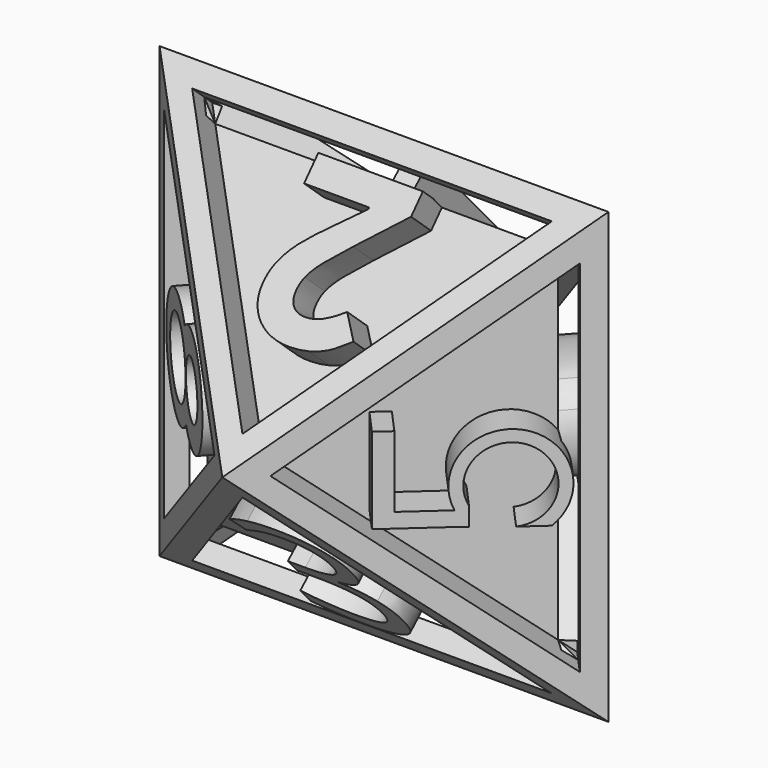
from build123d import *

# Parameters (mm, degrees)
F0_W      = 20
F0_H      = 20
F1_FACE_W = 20
F1_FACE_H = 20
F11_DEPTH = 1.5
F12_DEPTH = 1.5
F13_DEPTH = 1.5
F14_DEPTH = 1.5
F7_R      = 1.2292733426
F15_DEPTH = 1.5
F16_DEPTH = 1.5
F17_DEPTH = 1.5
F18_DEPTH = 1
F19_DEPTH = 1


# Not quite as in the source:
# - an extrude whose draft closes it to a point is written as a loft to that point
# - a feature names something its author has since deleted; it is built from what else it names


with BuildPart() as f1:
    # F0 (on Front) → F1 section 0
    with BuildSketch(Plane.XZ, mode=Mode.PRIVATE) as f1_s0:
        with Locations((-8.0479989899, 1.5718473494)):
            Rectangle(F0_W, F0_H)
    loft([f1_s0.sketch, Vertex(-8.0479989899, -9.004040443, 1.5718473494)], ruled=True)

    # F1_face (on face) → F2 section 0
    with BuildSketch(Plane(origin=(-8.0479989899, 0, 1.5718473494), x_dir=(1, 0, 0), z_dir=(0, 1, 0)), mode=Mode.PRIVATE) as f2_s0:
        Rectangle(F1_FACE_W, F1_FACE_H)
    loft([f2_s0.sketch, Vertex(-8.0479989899, 9.004040443, 1.5718473494)], ruled=True)

    # F8 (on face) → F11 (cut)
    with BuildSketch(Plane(origin=(0, -5.7542277794, 5.1811299644), x_dir=(1, 0, 0), z_dir=(0, -0.7431448255, 0.6691306064))):
        Polygon((-16.0589551992, 7.5995584789), (-8.0479989899, -3.1802463917), (-0.0370427807, 7.5995584789), align=None)
        with BuildLine():
            Line((-10.1255093079, 5.8311121626), (-10.1255093079, 7.0160687901))
            Line((-10.1255093079, 7.0160687901), (-5.470218449, 7.0160687901))
            Line((-5.470218449, 7.0160687901), (-5.470218449, 6.0366212456))
            Line((-5.470218449, 6.0366212456), (-7.1419838263, 4.3473657335))
            add(Edge.make_bspline(
                [(-7.1419838263, 4.3473657335), (-7.8853145521, 3.586544873), (-8.1126863035, 3.2928563608)],
                knots=[0, 0, 0, 1, 1, 1], degree=2))
            add(Edge.make_bspline(
                [(-8.1126863035, 3.2928563608), (-8.3400580549, 2.9991678486), (-8.4406263295, 2.7484759175)],
                knots=[0, 0, 0, 1, 1, 1], degree=2))
            add(Edge.make_bspline(
                [(-8.4406263295, 2.7484759175), (-8.5411946042, 2.4977839865), (-8.5411946042, 2.2296019207)],
                knots=[0, 0, 0, 1, 1, 1], degree=2))
            add(Edge.make_bspline(
                [(-8.5411946042, 2.2296019207), (-8.5411946042, 1.8287863333), (-8.3196528977, 1.6327510733)],
                knots=[0, 0, 0, 1, 1, 1], degree=2))
            add(Edge.make_bspline(
                [(-8.3196528977, 1.6327510733), (-8.0981111912, 1.4367158133), (-7.7293608508, 1.4367158133)],
                knots=[0, 0, 0, 1, 1, 1], degree=2))
            add(Edge.make_bspline(
                [(-7.7293608508, 1.4367158133), (-7.3431203756, 1.4367158133), (-6.9787425689, 1.614532183)],
                knots=[0, 0, 0, 1, 1, 1], degree=2))
            add(Edge.make_bspline(
                [(-6.9787425689, 1.614532183), (-6.6143647621, 1.7923485527), (-6.2179217084, 2.1202885787)],
                knots=[0, 0, 0, 1, 1, 1], degree=2))
            Line((-6.2179217084, 2.1202885787), (-5.4527283143, 1.2137165955))
            add(Edge.make_bspline(
                [(-5.4527283143, 1.2137165955), (-5.9439095977, 0.7939533622), (-6.2674770901, 0.6212382818)],
                knots=[0, 0, 0, 1, 1, 1], degree=2))
            add(Edge.make_bspline(
                [(-6.2674770901, 0.6212382818), (-6.5910445825, 0.4485232014), (-6.9736412796, 0.3552424829)],
                knots=[0, 0, 0, 1, 1, 1], degree=2))
            add(Edge.make_bspline(
                [(-6.9736412796, 0.3552424829), (-7.3562379767, 0.2619617643), (-7.8299291254, 0.2619617643)],
                knots=[0, 0, 0, 1, 1, 1], degree=2))
            add(Edge.make_bspline(
                [(-7.8299291254, 0.2619617643), (-8.4537439306, 0.2619617643), (-8.931807613, 0.4893335157)],
                knots=[0, 0, 0, 1, 1, 1], degree=2))
            add(Edge.make_bspline(
                [(-8.931807613, 0.4893335157), (-9.4098712955, 0.7167052671), (-9.6744095832, 1.1269946775)],
                knots=[0, 0, 0, 1, 1, 1], degree=2))
            add(Edge.make_bspline(
                [(-9.6744095832, 1.1269946775), (-9.9389478709, 1.5372840879), (-9.9389478709, 2.0649031521)],
                knots=[0, 0, 0, 1, 1, 1], degree=2))
            add(Edge.make_bspline(
                [(-9.9389478709, 2.0649031521), (-9.9389478709, 2.5254766998), (-9.7771641247, 2.9284785541)],
                knots=[0, 0, 0, 1, 1, 1], degree=2))
            add(Edge.make_bspline(
                [(-9.7771641247, 2.9284785541), (-9.6153803785, 3.3314804083), (-9.2757802626, 3.7548874198)],
                knots=[0, 0, 0, 1, 1, 1], degree=2))
            add(Edge.make_bspline(
                [(-9.2757802626, 3.7548874198), (-8.9361801467, 4.1782944312), (-8.0806210565, 4.9624354713)],
                knots=[0, 0, 0, 1, 1, 1], degree=2))
            Line((-8.0806210565, 4.9624354713), (-7.223604455, 5.7684391798))
            Line((-7.223604455, 5.7684391798), (-7.223604455, 5.8311121626))
            Line((-7.223604455, 5.8311121626), (-10.1255093079, 5.8311121626))
        make_face(mode=Mode.SUBTRACT)
    extrude(amount=-F11_DEPTH, mode=Mode.SUBTRACT)

    # F9 (on face) → F12 (cut)
    with BuildSketch(Plane(origin=(0.8739806721, -0.9706538721, 0), x_dir=(0.7431448255, 0.6691306064, 0), z_dir=(0.6691306064, -0.7431448255, 0))):
        Polygon((0.45061945, 9.5828035587), (-10.3291854207, 1.5718473494), (0.45061945, -6.4391088599), align=None)
        with BuildLine():
            Line((-6.7914770916, -0.6216760376), (-6.7914770916, 3.1999400918))
            Line((-6.7914770916, 3.1999400918), (-6.0100099072, 3.1999400918))
            Line((-6.0100099072, 3.1999400918), (-6.0100099072, 0.0335111318))
            Line((-6.0100099072, 0.0335111318), (-3.9149023546, 0.0335111318))
            ThreePointArc((-3.9149023546, 0.0335111318), (-1.5046868703, 3.1151424708), (-0.5219964927, -0.6716648932))
            Line((-0.5219964927, -0.6716648932), (-1.7677578144, -0.6716648932))
            ThreePointArc((-1.7677578144, -0.6716648932), (-1.1781497358, 2.4500116664), (-3.408615146, 0.1878166521))
            Line((-3.408615146, 0.1878166521), (-3.408615146, -0.6312971566))
            Line((-3.408615146, -0.6312971566), (-3.682563547, -0.6216760376))
            Line((-3.682563547, -0.6216760376), (-6.7914770916, -0.6216760376))
        make_face(mode=Mode.SUBTRACT)
    extrude(amount=-F12_DEPTH, mode=Mode.SUBTRACT)

    # F10 (on face) → F13 (cut)
    with BuildSketch(Plane(origin=(0, -4.1909911743, -3.7735854029), x_dir=(1, 0, 0), z_dir=(0, -0.7431448255, -0.6691306064))):
        Polygon((-0.0370427807, -5.2633380306), (-8.0479989899, 5.51646684), (-16.0589551992, -5.2633380306), align=None)
        with BuildLine():
            add(Edge.make_bspline(
                [(-6.2778853712, 2.3209247428), (-5.6446293929, 1.7983598502), (-5.6446293929, 0.8870890521)],
                knots=[0, 0, 0, 1, 1, 1], degree=2))
            add(Edge.make_bspline(
                [(-5.6446293929, 0.8870890521), (-5.6446293929, 0.1354193543), (-6.0659419747, -0.3416678055)],
                knots=[0, 0, 0, 1, 1, 1], degree=2))
            add(Edge.make_bspline(
                [(-6.0659419747, -0.3416678055), (-6.4872545565, -0.8187549653), (-7.2595179446, -0.9800722064)],
                knots=[0, 0, 0, 1, 1, 1], degree=2))
            Line((-7.2595179446, -0.9800722064), (-7.2595179446, -1.022975728))
            add(Edge.make_bspline(
                [(-7.2595179446, -1.022975728), (-6.3156404702, -1.1396733066), (-5.8600050712, -1.6227669594)],
                knots=[0, 0, 0, 1, 1, 1], degree=2))
            add(Edge.make_bspline(
                [(-5.8600050712, -1.6227669594), (-5.4043696722, -2.1058606123), (-5.4043696722, -2.8884208456)],
                knots=[0, 0, 0, 1, 1, 1], degree=2))
            add(Edge.make_bspline(
                [(-5.4043696722, -2.8884208456), (-5.4043696722, -4.0090608289), (-6.1817814829, -4.6131424125)],
                knots=[0, 0, 0, 1, 1, 1], degree=2))
            add(Edge.make_bspline(
                [(-6.1817814829, -4.6131424125), (-6.9591932937, -5.2172239962), (-8.3904547731, -5.2172239962)],
                knots=[0, 0, 0, 1, 1, 1], degree=2))
            add(Edge.make_bspline(
                [(-8.3904547731, -5.2172239962), (-9.0134139062, -5.2172239962), (-9.5308303763, -5.1228362487)],
                knots=[0, 0, 0, 1, 1, 1], degree=2))
            add(Edge.make_bspline(
                [(-9.5308303763, -5.1228362487), (-10.0482468464, -5.0284485013), (-10.5356308513, -4.7933372031)],
                knots=[0, 0, 0, 1, 1, 1], degree=2))
            Line((-10.5356308513, -4.7933372031), (-10.5356308513, -3.945563617))
            add(Edge.make_bspline(
                [(-10.5356308513, -3.945563617), (-10.0259370151, -4.1978363238), (-9.4493136853, -4.3291210998)],
                knots=[0, 0, 0, 1, 1, 1], degree=2))
            add(Edge.make_bspline(
                [(-9.4493136853, -4.3291210998), (-8.8726903555, -4.4604058758), (-8.3578480967, -4.4604058758)],
                knots=[0, 0, 0, 1, 1, 1], degree=2))
            add(Edge.make_bspline(
                [(-8.3578480967, -4.4604058758), (-6.3259373154, -4.4604058758), (-6.3259373154, -2.8678271553)],
                knots=[0, 0, 0, 1, 1, 1], degree=2))
            add(Edge.make_bspline(
                [(-6.3259373154, -2.8678271553), (-6.3259373154, -1.4399979576), (-8.5672172819, -1.4399979576)],
                knots=[0, 0, 0, 1, 1, 1], degree=2))
            Line((-8.5672172819, -1.4399979576), (-9.3394806701, -1.4399979576))
            Line((-9.3394806701, -1.4399979576), (-9.3394806701, -0.6745991329))
            Line((-9.3394806701, -0.6745991329), (-8.5569204368, -0.6745991329))
            add(Edge.make_bspline(
                [(-8.5569204368, -0.6745991329), (-7.6405012161, -0.6745991329), (-7.1042071966, -0.2695898893)],
                knots=[0, 0, 0, 1, 1, 1], degree=2))
            add(Edge.make_bspline(
                [(-7.1042071966, -0.2695898893), (-6.567913177, 0.1354193543), (-6.567913177, 0.8544823757)],
                knots=[0, 0, 0, 1, 1, 1], degree=2))
            add(Edge.make_bspline(
                [(-6.567913177, 0.8544823757), (-6.567913177, 1.4276734238), (-6.961767505, 1.7554563286)],
                knots=[0, 0, 0, 1, 1, 1], degree=2))
            add(Edge.make_bspline(
                [(-6.961767505, 1.7554563286), (-7.3556218329, 2.0832392333), (-8.0317813328, 2.0832392333)],
                knots=[0, 0, 0, 1, 1, 1], degree=2))
            add(Edge.make_bspline(
                [(-8.0317813328, 2.0832392333), (-8.5466235916, 2.0832392333), (-9.0022589906, 1.943373753)],
                knots=[0, 0, 0, 1, 1, 1], degree=2))
            add(Edge.make_bspline(
                [(-9.0022589906, 1.943373753), (-9.4578943896, 1.8035082727), (-10.0430984238, 1.4276734238)],
                knots=[0, 0, 0, 1, 1, 1], degree=2))
            Line((-10.0430984238, 1.4276734238), (-10.4927273298, 2.0283227257))
            add(Edge.make_bspline(
                [(-10.4927273298, 2.0283227257), (-10.0104917474, 2.4093059972), (-9.3806680508, 2.6263978164)],
                knots=[0, 0, 0, 1, 1, 1], degree=2))
            add(Edge.make_bspline(
                [(-9.3806680508, 2.6263978164), (-8.7508443542, 2.8434896355), (-8.0523750232, 2.8434896355)],
                knots=[0, 0, 0, 1, 1, 1], degree=2))
            add(Edge.make_bspline(
                [(-8.0523750232, 2.8434896355), (-6.9111413495, 2.8434896355), (-6.2778853712, 2.3209247428)],
                knots=[0, 0, 0, 1, 1, 1], degree=2))
        make_face(mode=Mode.SUBTRACT)
    extrude(amount=-F13_DEPTH, mode=Mode.SUBTRACT)

    # F7 (on face) → F14 (cut)
    with BuildSketch(Plane(origin=(-8.0807346952, -8.9745650815, 0), x_dir=(0.7431448255, -0.6691306064, 0), z_dir=(-0.6691306064, -0.7431448255, 0))):
        Polygon((-12.4122770596, -6.4391088599), (-1.632472189, 1.5718473494), (-12.4122770596, 9.5828035587), align=None)
        with BuildLine():
            ThreePointArc((-8.0010479185, 3.3852743433), (-4.2277937132, 1.7916034584), (-7.7158939093, -0.3555786971))
            ThreePointArc((-7.7158939093, -0.3555786971), (-11.95616225, 1.2024931008), (-8.0010479185, 3.3852743433))
        make_face(mode=Mode.SUBTRACT)
        with BuildLine():
            ThreePointArc((-7.835039689, 1.3912107131), (-7.8362300165, 1.4537861947), (-7.8397992768, 1.516271138))
            ThreePointArc((-7.8397992768, 1.516271138), (-11.1246308448, 1.3286352316), (-7.835039689, 1.3912107131))
        make_face()
    extrude(amount=-F14_DEPTH, mode=Mode.SUBTRACT)

    # F7 (on face) → F15 (cut)
    with BuildSketch(Plane(origin=(-8.0807346952, -8.9745650815, 0), x_dir=(0.7431448255, -0.6691306064, 0), z_dir=(-0.6691306064, -0.7431448255, 0))):
        with Locations((-6.5249288455, 1.616499736)):
            Circle(F7_R)
    extrude(amount=-F15_DEPTH, mode=Mode.SUBTRACT)

    # F4 (on face) → F16 (cut)
    with BuildSketch(Plane(origin=(0.8739806721, 0.9706538721, 0), x_dir=(-0.7431448255, 0.6691306064, 0), z_dir=(0.6691306064, 0.7431448255, 0))):
        Polygon((-0.45061945, -6.4391088599), (10.3291854207, 1.5718473494), (-0.45061945, 9.5828035587), align=None)
        with BuildLine():
            add(Edge.make_bspline(
                [(1.6306424047, 3.545827145), (2.2208165521, 3.8140285075), (3.053617849, 3.8140285075)],
                knots=[0, 0, 0, 1, 1, 1], degree=2))
            add(Edge.make_bspline(
                [(3.053617849, 3.8140285075), (4.8320092799, 3.8140285075), (5.7008767747, 3.0618843441)],
                knots=[0, 0, 0, 1, 1, 1], degree=2))
            add(Edge.make_bspline(
                [(5.7008767747, 3.0618843441), (6.5697442695, 2.3097401806), (6.5697442695, 0.8093863481)],
                knots=[0, 0, 0, 1, 1, 1], degree=2))
            add(Edge.make_bspline(
                [(6.5697442695, 0.8093863481), (6.5697442695, 0.297902087), (6.5081038586, 0.0067495076)],
                knots=[0, 0, 0, 1, 1, 1], degree=2))
            Line((6.5081038586, 0.0067495076), (5.4956273212, 0.0067495076))
            add(Edge.make_bspline(
                [(5.4956273212, 0.0067495076), (5.5782517018, 0.3713459809), (5.5782517018, 0.7280734656)],
                knots=[0, 0, 0, 1, 1, 1], degree=2))
            add(Edge.make_bspline(
                [(5.5782517018, 0.7280734656), (5.5782517018, 1.3798880239), (5.381526986, 1.791698429)],
                knots=[0, 0, 0, 1, 1, 1], degree=2))
            add(Edge.make_bspline(
                [(5.381526986, 1.791698429), (5.1848022702, 2.2035088341), (4.7992218272, 2.4081025385)],
                knots=[0, 0, 0, 1, 1, 1], degree=2))
            add(Edge.make_bspline(
                [(4.7992218272, 2.4081025385), (4.4136413843, 2.612696243), (3.7054324074, 2.6494181899)],
                knots=[0, 0, 0, 1, 1, 1], degree=2))
            Line((3.7054324074, 2.6494181899), (3.7054324074, 2.5969582657))
            add(Edge.make_bspline(
                [(3.7054324074, 2.5969582657), (4.4018379013, 2.190393853), (4.4018379013, 1.2972636433)],
                knots=[0, 0, 0, 1, 1, 1], degree=2))
            add(Edge.make_bspline(
                [(4.4018379013, 1.2972636433), (4.4018379013, 0.4946268028), (3.8975668798, 0.0395369602)],
                knots=[0, 0, 0, 1, 1, 1], degree=2))
            add(Edge.make_bspline(
                [(3.8975668798, 0.0395369602), (3.3932958583, -0.4155528823), (2.5041001428, -0.4155528823)],
                knots=[0, 0, 0, 1, 1, 1], degree=2))
            add(Edge.make_bspline(
                [(2.5041001428, -0.4155528823), (1.5453950278, -0.4155528823), (0.9853853368, 0.1254400861)],
                knots=[0, 0, 0, 1, 1, 1], degree=2))
            add(Edge.make_bspline(
                [(0.9853853368, 0.1254400861), (0.4253756458, 0.6664330546), (0.4253756458, 1.6251381696)],
                knots=[0, 0, 0, 1, 1, 1], degree=2))
            add(Edge.make_bspline(
                [(0.4253756458, 1.6251381696), (0.4253756458, 2.2887562109), (0.7329219515, 2.7831909967)],
                knots=[0, 0, 0, 1, 1, 1], degree=2))
            add(Edge.make_bspline(
                [(0.7329219515, 2.7831909967), (1.0404682572, 3.2776257824), (1.6306424047, 3.545827145)],
                knots=[0, 0, 0, 1, 1, 1], degree=2))
        make_face(mode=Mode.SUBTRACT)
        with BuildLine():
            add(Edge.make_bspline(
                [(1.7742514472, 2.2999039448), (1.4378521832, 2.0435060652), (1.4378521832, 1.6500566336)],
                knots=[0, 0, 0, 1, 1, 1], degree=2))
            add(Edge.make_bspline(
                [(1.4378521832, 1.6500566336), (1.4378521832, 1.2448037191), (1.7106437891, 1.0270950336)],
                knots=[0, 0, 0, 1, 1, 1], degree=2))
            add(Edge.make_bspline(
                [(1.7106437891, 1.0270950336), (1.983435395, 0.8093863481), (2.4870506675, 0.8093863481)],
                knots=[0, 0, 0, 1, 1, 1], degree=2))
            add(Edge.make_bspline(
                [(2.4870506675, 0.8093863481), (2.9264025328, 0.8093863481), (3.178210169, 1.0126685544)],
                knots=[0, 0, 0, 1, 1, 1], degree=2))
            add(Edge.make_bspline(
                [(3.178210169, 1.0126685544), (3.4300178052, 1.2159507608), (3.4300178052, 1.6251381696)],
                knots=[0, 0, 0, 1, 1, 1], degree=2))
            add(Edge.make_bspline(
                [(3.4300178052, 1.6251381696), (3.4300178052, 2.0107186126), (3.1801774162, 2.2835102185)],
                knots=[0, 0, 0, 1, 1, 1], degree=2))
            add(Edge.make_bspline(
                [(3.1801774162, 2.2835102185), (2.9303370271, 2.5563018244), (2.5985280064, 2.5563018244)],
                knots=[0, 0, 0, 1, 1, 1], degree=2))
            add(Edge.make_bspline(
                [(2.5985280064, 2.5563018244), (2.1106507112, 2.5563018244), (1.7742514472, 2.2999039448)],
                knots=[0, 0, 0, 1, 1, 1], degree=2))
        make_face()
    extrude(amount=-F16_DEPTH, mode=Mode.SUBTRACT)

    # F3 (on face) → F17 (cut)
    with BuildSketch(Plane(origin=(0, 5.7542277794, 5.1811299644), x_dir=(-1, 0, 0), z_dir=(0, 0.7431448255, 0.6691306064))):
        Polygon((0.0370427807, 7.5995584789), (8.0479989899, -3.1802463917), (16.0589551992, 7.5995584789), align=None)
        Polygon((7.9576568678, 0.6158080068), (9.2136384919, 0.6158080068), (9.1912923381, 0), (7.9576568678, -1.1053429917), (6.9978768006, -1.1053429917), (6.9978768006, 6.7507135682), (7.9576568678, 6.7507135682), align=None, mode=Mode.SUBTRACT)
    extrude(amount=-F17_DEPTH, mode=Mode.SUBTRACT)

    # F6 (on face) → F18 (cut)
    with BuildSketch(Plane(origin=(-8.0807346952, 8.9745650815, 0), x_dir=(-0.7431448255, -0.6691306064, 0), z_dir=(-0.6691306064, 0.7431448255, 0))):
        Polygon((12.4122770596, 9.5828035587), (1.632472189, 1.5718473494), (12.4122770596, -6.4391088599), align=None)
        Polygon((6.6518909298, -0.8224349432), (5.5364738218, -0.8730660775), (5.5364738218, 4.1275592521), (12.1340155602, 3.0015249307), (12.1340155602, 1.7575944075), (6.6518909298, 2.7529795188), align=None, mode=Mode.SUBTRACT)
    extrude(amount=-F18_DEPTH, mode=Mode.SUBTRACT)

    # F5 (on face) → F19 (cut)
    with BuildSketch(Plane(origin=(0, 4.1909911743, -3.7735854029), x_dir=(-1, 0, 0), z_dir=(0, 0.7431448255, -0.6691306064))):
        Polygon((16.0589551992, -5.2633380306), (8.0479989899, 5.51646684), (0.0370427807, -5.2633380306), align=None)
        Polygon((10.5934113821, -2.0774938067), (10.5934113821, -3.341090436), (9.6667738539, -3.341090436), (9.6667738539, -4.93659178), (8.0763268965, -4.93659178), (8.0763268965, -3.341090436), (4.7909756603, -3.341090436), (4.7909756603, -2.2089078562), (8.1673058538, 2.7612388858), (9.6667738539, 2.7612388858), (9.6667738539, -2.0774938067), align=None, mode=Mode.SUBTRACT)
        with BuildLine():
            Line((6.2230518402, -2.0774938067), (8.0763268965, -2.0774938067))
            Line((8.0763268965, -2.0774938067), (8.0763268965, -0.7717772898))
            add(Edge.make_bspline(
                [(8.0763268965, -0.7717772898), (8.0763268965, -0.4449269617), (8.1032836246, 0.1759201822)],
                knots=[0, 0, 0, 1, 1, 1], degree=2))
            add(Edge.make_bspline(
                [(8.1032836246, 0.1759201822), (8.1302403527, 0.7967673261), (8.1454035122, 0.8978550564)],
                knots=[0, 0, 0, 1, 1, 1], degree=2))
            Line((8.1454035122, 0.8978550564), (8.1032836246, 0.8978550564))
            add(Edge.make_bspline(
                [(8.1032836246, 0.8978550564), (7.9078473459, 0.4648626114), (7.634910474, 0.0554573035)],
                knots=[0, 0, 0, 1, 1, 1], degree=2))
            Line((7.634910474, 0.0554573035), (6.2230518402, -2.0774938067))
        make_face()
    extrude(amount=-F19_DEPTH, mode=Mode.SUBTRACT)


solid = f1.part
